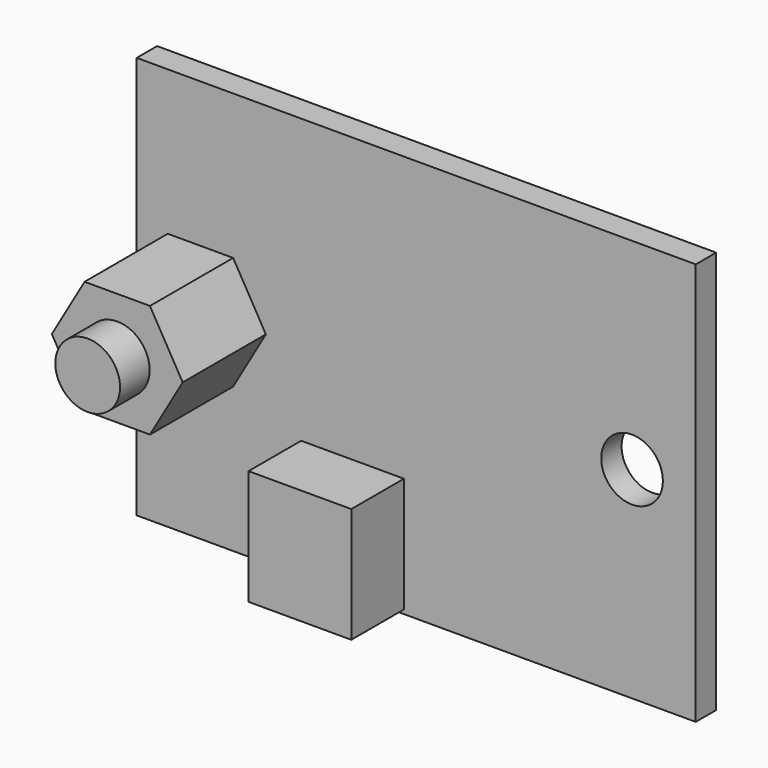
from build123d import *

# Parameters (mm, degrees)
F0_W     = 34.544
F0_H     = 24.892
F0_R     = 1.905
F1_DEPTH = 1.5748
F2_W     = 6.35
F2_H     = 7.112
F3_DEPTH = 4.064
F4_R     = 2
F5_DEPTH = 8
F6_START = 7
F6_DEPTH = 3.287


with BuildPart() as f1:
    # F0 (on Front) → F1 (new body)
    with BuildSketch(Plane.XZ):
        Rectangle(F0_W, F0_H)
        with Locations((-13.335, 0)):
            Circle(F0_R, mode=Mode.SUBTRACT)
        with Locations((13.335, 0)):
            Circle(F0_R, mode=Mode.SUBTRACT)
    extrude(amount=F1_DEPTH)

    # F2 (on face) → F3 (join)
    with BuildSketch(Plane.XZ.offset(1.5748)):
        with Locations((-3.937, -8.636)):
            Rectangle(F2_W, F2_H)
    extrude(amount=F3_DEPTH)


with BuildPart() as f5:
    # F4 (on Front) → F5 (new body)
    with BuildSketch(Plane.XZ):
        Polygon((-11.3142740578, -3.5), (-9.2935481157, 0), (-11.3142740578, 3.5), (-15.3557259422, 3.5), (-17.3764518843, 0), (-15.3557259422, -3.5), align=None)
        with Locations((-13.335, 0)):
            Circle(F4_R, mode=Mode.SUBTRACT)
    extrude(amount=F5_DEPTH)

    # F4 (on Front) → F6 (join)
    with BuildSketch(Plane.XZ.offset(F6_START)):
        with Locations((-13.335, 0)):
            Circle(F4_R)
    extrude(amount=F6_DEPTH)


solid = Compound([f1.part, f5.part])
